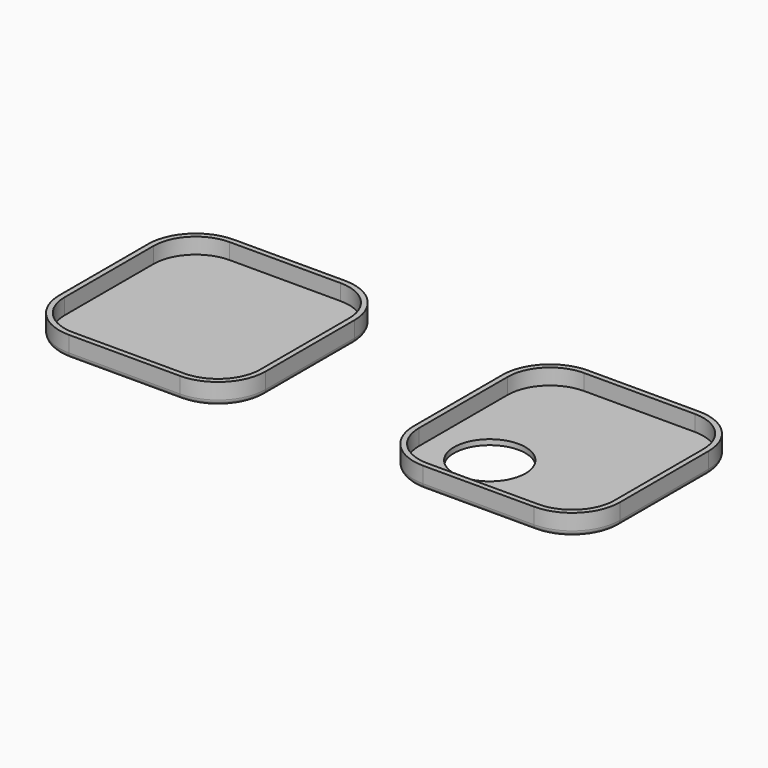
from build123d import *

# Parameters (mm, degrees)
F0_W         = 37
F0_H         = 37
F1_DEPTH     = 3
F2_R         = 8
F3_T         = 1
F4_T1_DEPTH  = 21
F4_T3_DEPTH  = 21
F4_T6_ANGLE  = 90
F4_T8_ANGLE  = 90
F4_T10_ANGLE = 90
F4_T12_ANGLE = 90
F6_R         = 6.75
F7_DEPTH     = 1


# Not quite as in the source:
# - a fillet or chamfer that OpenCascade refuses, or shapes differently, is made with other operations: its cross-section is extruded or revolved along the edge and cut away or added


with BuildPart() as f1:
    # F0 (on Top) → F1 (new body)
    with BuildSketch(Plane.XY):
        with Locations((33.5, 0)):
            Rectangle(F0_W, F0_H)
    extrude(amount=F1_DEPTH)

    # F2
    f2_edges = [f1.edges().sort_by_distance(p)[0] for p in [
        (15, 18.5, 1.5),
        (52, 18.5, 1.5),
        (52, -18.5, 1.5),
        (15, -18.5, 1.5),
    ]]
    fillet(f2_edges, radius=F2_R)

    # F3
    f3_openings = [f1.faces().sort_by_distance(p)[0] for p in [
        (33.5, 0, 3),
    ]]
    offset(amount=F3_T, openings=f3_openings, kind=Kind.INTERSECTION)

    # F4: fillet of radius 1 on 8 edges, made by hand

    # F4_s2 → F4_t1 (cut)
    with BuildSketch(Plane.YZ.offset(23)):
        with BuildLine():
            ThreePointArc((19.5, 0), (19.2071067812, -0.7071067812), (18.5, -1))
            Line((18.5, -1), (19.5, -1))
            Line((19.5, -1), (19.5, 0))
        make_face()
        with BuildLine():
            ThreePointArc((-18.5, -1), (-19.2071067812, -0.7071067812), (-19.5, 0))
            Line((-19.5, 0), (-19.5, -1))
            Line((-19.5, -1), (-18.5, -1))
        make_face()
    extrude(amount=F4_T1_DEPTH, mode=Mode.SUBTRACT)

    # F4_s4 → F4_t3 (cut)
    with BuildSketch(Plane.XZ.offset(-10.5)):
        with BuildLine():
            ThreePointArc((15, -1), (14.2928932188, -0.7071067812), (14, 0))
            Line((14, 0), (14, -1))
            Line((14, -1), (15, -1))
        make_face()
        with BuildLine():
            ThreePointArc((52, -1), (52.7071067812, -0.7071067812), (53, 0))
            Line((53, 0), (53, -1))
            Line((53, -1), (52, -1))
        make_face()
    extrude(amount=F4_T3_DEPTH, mode=Mode.SUBTRACT)

    # F4_s5 → F4_t6 (revolve, cut)
    with BuildSketch(Plane.XZ.offset(-10.5)):
        with BuildLine():
            ThreePointArc((52, -1), (52.7071067812, -0.7071067812), (53, 0))
            Line((53, 0), (53, -1))
            Line((53, -1), (52, -1))
        make_face()
    revolve(axis=Axis((44, 10.5, -1), (0, 0, 1)), revolution_arc=F4_T6_ANGLE, mode=Mode.SUBTRACT)

    # F4_s7 → F4_t8 (revolve, cut)
    with BuildSketch(Plane.YZ.offset(23)):
        with BuildLine():
            ThreePointArc((18.5, -1), (19.2071067812, -0.7071067812), (19.5, 0))
            Line((19.5, 0), (19.5, -1))
            Line((19.5, -1), (18.5, -1))
        make_face()
    revolve(axis=Axis((23, 10.5, -1), (0, 0, 1)), revolution_arc=F4_T8_ANGLE, mode=Mode.SUBTRACT)

    # F4_s9 → F4_t10 (revolve, cut)
    with BuildSketch(Plane.XZ.offset(10.5)):
        with BuildLine():
            ThreePointArc((15, -1), (14.2928932188, -0.7071067812), (14, 0))
            Line((14, 0), (14, -1))
            Line((14, -1), (15, -1))
        make_face()
    revolve(axis=Axis((23, -10.5, -1), (0, 0, 1)), revolution_arc=F4_T10_ANGLE, mode=Mode.SUBTRACT)

    # F4_s11 → F4_t12 (revolve, cut)
    with BuildSketch(Plane.YZ.offset(44)):
        with BuildLine():
            ThreePointArc((-18.5, -1), (-19.2071067812, -0.7071067812), (-19.5, 0))
            Line((-19.5, 0), (-19.5, -1))
            Line((-19.5, -1), (-18.5, -1))
        make_face()
    revolve(axis=Axis((44, -10.5, -1), (0, 0, 1)), revolution_arc=F4_T12_ANGLE, mode=Mode.SUBTRACT)


with BuildPart() as f5_1:
    # F5: instance of F1
    add(f1.part.mirror(Plane.YZ))


with BuildPart() as f1_1:
    add(f1.part)

    # F6 (on face) → F7 (cut, through all)
    with BuildSketch(Plane.XY):
        with Locations((26, -7.5)):
            Circle(F6_R)
    extrude(amount=-F7_DEPTH, mode=Mode.SUBTRACT)


solid = Compound([f5_1.part, f1_1.part])
